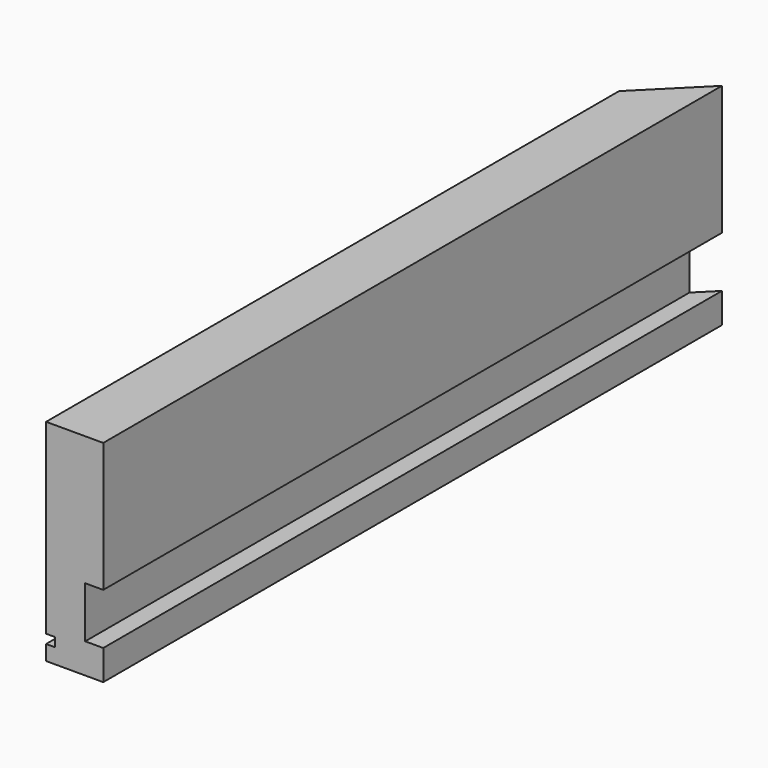
from build123d import *

# Parameters (mm, degrees)
F0_W        = 257
F0_H        = 70
F1_DEPTH    = 19
F2_W        = 3
F2_H        = 3
F3_DEPTH    = 257.001
F4_W        = 6
F4_H        = 17
F5_DEPTH    = 257.001
F6_T1_DEPTH = 159.7239535427


# Not quite as in the source:
# - a fillet or chamfer that OpenCascade refuses, or shapes differently, is made with other operations: its cross-section is extruded or revolved along the edge and cut away or added


with BuildPart() as f1:
    # F0 (on Right) → F1 (new body)
    with BuildSketch(Plane.YZ):
        with Locations((-128.5, 35)):
            Rectangle(F0_W, F0_H)
    extrude(amount=F1_DEPTH)

    # F2 (on face) → F3 (cut, through all)
    with BuildSketch(Plane.XZ.offset(257)):
        with Locations((1.5, 6.5)):
            Rectangle(F2_W, F2_H)
    extrude(amount=-F3_DEPTH, mode=Mode.SUBTRACT)

    # F4 (on face) → F5 (cut, through all)
    with BuildSketch(Plane.XZ.offset(257)):
        with Locations((16, 18.5)):
            Rectangle(F4_W, F4_H)
    extrude(amount=-F5_DEPTH, mode=Mode.SUBTRACT)

    # F6: chamfer of 19 on 1 edges, made by hand

    # F6_s2 → F6_t1 (cut)
    with BuildSketch(Plane.XY.offset(-40.8619767714)):
        Polygon((19, 0), (0, -19), (0, 0), align=None)
    extrude(amount=F6_T1_DEPTH, mode=Mode.SUBTRACT)


solid = f1.part
